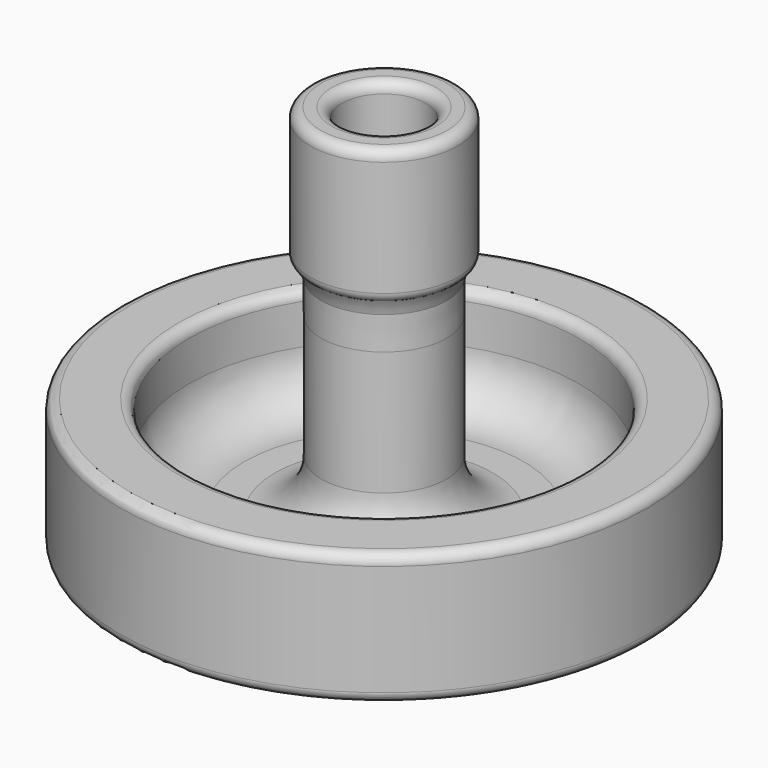
from build123d import *

# Parameters (mm, degrees)
F3_R = 0.5


# Not quite as in the source:
# - a fillet or chamfer that OpenCascade refuses, or shapes differently, is made with other operations: its cross-section is extruded or revolved along the edge and cut away or added
# - a feature names something its author has since deleted; it is built from what else it names


with BuildPart() as f1:
    # F0 (on Front) → F1 (revolve)
    with BuildSketch(Plane.XZ):
        with BuildLine():
            Line((-12.2, 0), (-6.35, 0))
            ThreePointArc((-6.35, 0), (-3.6810616685, -0.5842717783), (-1.5003500059, -2.2302067626))
            ThreePointArc((-1.5003500059, -2.2302067626), (-1.292996294, -0.7904112116), (0, -0.1239523798))
            Line((0, -0.1239523798), (0, 0))
            Line((0, 0), (0, 4.6583339572))
            Line((0, 4.6583339572), (-1.5205304027, 4.6583339572))
            ThreePointArc((-1.5205304027, 4.6583339572), (-1.8740837933, 4.8047805666), (-2.0205304027, 5.1583339572))
            Line((-2.0205304027, 5.1583339572), (-2.0205304027, 18.7134853154))
            Line((-2.0205304027, 18.7134853154), (-3.0250614509, 18.7134853154))
            Line((-3.0250614509, 18.7134853154), (-3.5481122322, 18.7134853154))
            Line((-3.5481122322, 18.7134853154), (-3.5481122322, 12.2134853154))
            Line((-3.5481122322, 12.2134853154), (-3.2865868416, 12.2134853154))
            ThreePointArc((-3.2865868416, 12.2134853154), (-3.1265563478, 11.8601003085), (-3.0236392793, 11.4860698297))
            Line((-3.0236392793, 11.4860698297), (-3.0205304027, 9.8959347233))
            Line((-3.0205304027, 9.8959347233), (-3.0205304027, 3.925))
            ThreePointArc((-3.0205304027, 3.925), (-3.6626216951, 2.2779224085), (-5.2500669844, 1.5))
            Line((-5.2500669844, 1.5), (-6.7232404836, 1.5))
            ThreePointArc((-6.7232404836, 1.5), (-8.5932958155, 2.1254805036), (-9.3995602801, 3.925))
            Line((-9.3995602801, 3.925), (-9.3995602801, 5.85))
            ThreePointArc((-9.3995602801, 5.85), (-9.5460068896, 6.2035533906), (-9.8995602801, 6.35))
            Line((-9.8995602801, 6.35), (-12.2, 6.35))
            ThreePointArc((-12.2, 6.35), (-12.5535533906, 6.2035533906), (-12.7, 5.85))
            Line((-12.7, 5.85), (-12.7, 0.5))
            ThreePointArc((-12.7, 0.5), (-12.5535533906, 0.1464466094), (-12.2, 0))
        make_face()
    revolve(axis=Axis((0, 0, 3.175), (0, 0, 1)))

    # F2: fillet of radius 0.5 on 2 edges, made by hand

    # F2_s1 → F2_t2 (revolve, cut)
    with BuildSketch(Plane.XZ):
        with BuildLine():
            ThreePointArc((-3.0481122322, 18.7134853154), (-3.4016656228, 18.567038706), (-3.5481122322, 18.2134853154))
            Line((-3.5481122322, 18.2134853154), (-3.5581122322, 18.2134853154))
            Line((-3.5581122322, 18.2134853154), (-3.5581122322, 18.7234853154))
            Line((-3.5581122322, 18.7234853154), (-3.0481122322, 18.7234853154))
            Line((-3.0481122322, 18.7234853154), (-3.0481122322, 18.7134853154))
        make_face()
    revolve(axis=Axis((0, 0, 18.7134853154), (0, 0, 1)), mode=Mode.SUBTRACT)

    # F2_s3 → F2_t4 (revolve, cut)
    with BuildSketch(Plane.XZ):
        with BuildLine():
            ThreePointArc((-3.2865868416, 12.2134853154), (-3.4777849592, 12.3972529753), (-3.5481122322, 12.6529507415))
            Line((-3.5481122322, 12.6529507415), (-3.5581122322, 12.6529507415))
            Line((-3.5581122322, 12.6529507415), (-3.5581122322, 12.2134853154))
            Line((-3.5581122322, 12.2134853154), (-3.5481122322, 12.2034853154))
            ThreePointArc((-3.5481122322, 12.2034853154), (-3.4173495369, 12.2034853154), (-3.2913563338, 12.2046960069))
            Line((-3.2913563338, 12.2046960069), (-3.2865868416, 12.2134853154))
        make_face()
    revolve(axis=Axis((0, 0, 12.2134853154), (0, 0, 1)), mode=Mode.SUBTRACT)

    # F3
    f3_edges = [f1.edges().sort_by_distance(p)[0] for p in [
        (2.02053, 0, 18.713485),
    ]]
    fillet(f3_edges, radius=F3_R)


solid = f1.part
